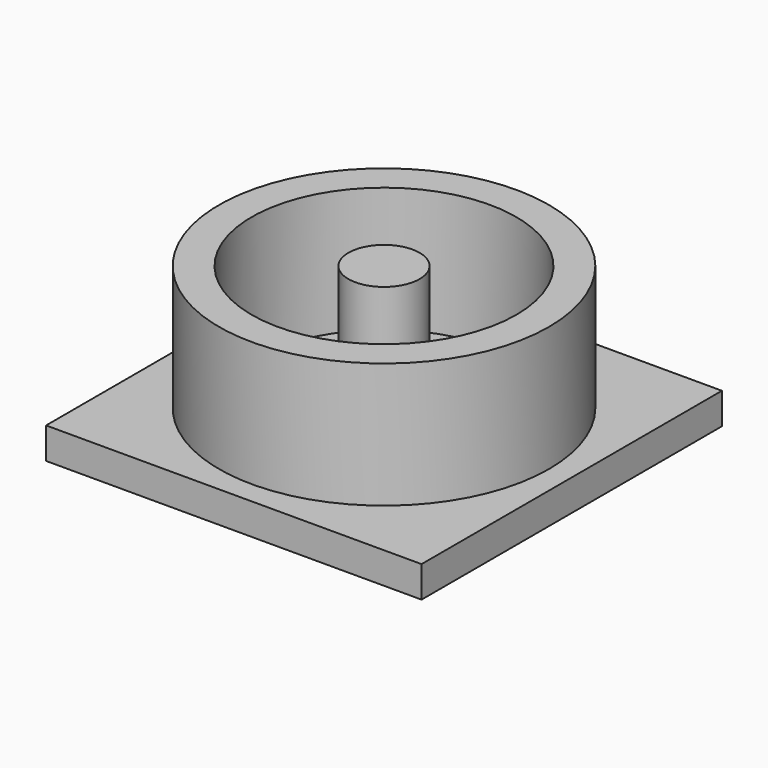
from build123d import *

# Parameters (mm, degrees)
F0_W     = 30
F0_H     = 30
F1_DEPTH = 2.5
F2_R     = 2.8452020341
F3_DEPTH = 12.5
F4_R     = 13.1863944163
F4_R_2   = 10.5757052103
F5_DEPTH = 12.5


# Not quite as in the source:
# - a feature names something its author has since deleted; it is built from what else it names


with BuildPart() as f1:
    # F0 (on Top) → F1 (new body)
    with BuildSketch(Plane.XY):
        Rectangle(F0_W, F0_H)
    extrude(amount=F1_DEPTH)

    # F2 (on Top) → F3 (join)
    with BuildSketch(Plane.XY):
        Circle(F2_R)
    extrude(amount=F3_DEPTH)

    # F4 (on Top) → F5 (join)
    with BuildSketch(Plane.XY):
        Circle(F4_R)
        Circle(F4_R_2, mode=Mode.SUBTRACT)
    extrude(amount=F5_DEPTH)


solid = f1.part
